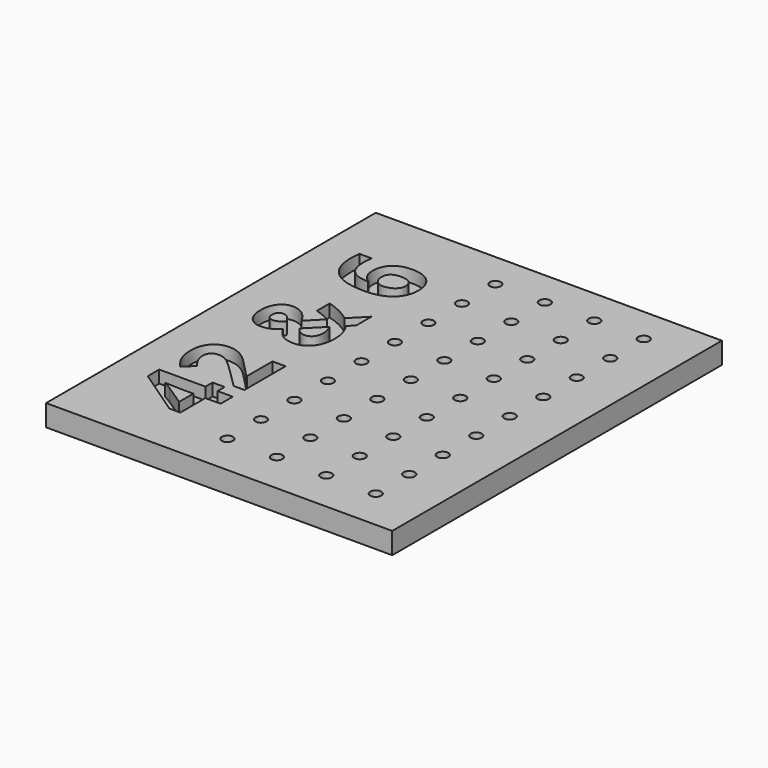
from build123d import *

# Parameters (mm, degrees)
F0_W         = 42
F0_H         = 50
F1_DEPTH     = 2.6
F2_TEXT_SIZE = 12.5
F3_DEPTH     = 1.5
F4_R         = 0.675
F5_DEPTH     = 2.6


# Not quite as in the source:
# - Text() gives the source's letters only with a copy of the font that has no kerning and outlines rounded to 1/6400 em; it was checked with that copy


with BuildPart() as f1:
    # F0 (on Top) → F1 (new body)
    with BuildSketch(Plane.XY):
        with Locations((-22.1587231159, 3.3350909071)):
            Rectangle(F0_W, F0_H)
    extrude(amount=F1_DEPTH)

    # F2 (on face) → F3 (cut)
    with BuildSketch(Plane.XY.offset(2.6)):
        with Locations(Location((-30.1587231159, -15.4649090929), (0, 0, 90))):
            Text('42 & 6', F2_TEXT_SIZE, font='Open Sans', font_style=FontStyle.BOLD, text_align=(TextAlign.LEFT, TextAlign.BOTTOM))
    extrude(amount=-F3_DEPTH, mode=Mode.SUBTRACT)

    # F4 (on face) → F5 (cut, through all)
    with BuildSketch(Plane.XY.offset(2.6)):
        with Locations((-25.1587231159, -16.6649090929)):
            Circle(F4_R)
        with Locations((-25.1587231159, -11.5849090929)):
            Circle(F4_R)
        with Locations((-25.1587231159, -6.5049090929)):
            Circle(F4_R)
        with Locations((-25.1587231159, -1.4249090929)):
            Circle(F4_R)
        with Locations((-25.1587231159, 3.6550909071)):
            Circle(F4_R)
        with Locations((-25.1587231159, 8.7350909071)):
            Circle(F4_R)
        with Locations((-25.1587231159, 13.8150909071)):
            Circle(F4_R)
        with Locations((-25.1587231159, 18.8950909071)):
            Circle(F4_R)
        with Locations((-19.1587231159, -16.6649090929)):
            Circle(F4_R)
        with Locations((-19.1587231159, -11.5849090929)):
            Circle(F4_R)
        with Locations((-19.1587231159, -6.5049090929)):
            Circle(F4_R)
        with Locations((-19.1587231159, -1.4249090929)):
            Circle(F4_R)
        with Locations((-19.1587231159, 3.6550909071)):
            Circle(F4_R)
        with Locations((-19.1587231159, 8.7350909071)):
            Circle(F4_R)
        with Locations((-19.1587231159, 13.8150909071)):
            Circle(F4_R)
        with Locations((-19.1587231159, 18.8950909071)):
            Circle(F4_R)
        with Locations((-13.1587231159, -16.6649090929)):
            Circle(F4_R)
        with Locations((-13.1587231159, -11.5849090929)):
            Circle(F4_R)
        with Locations((-13.1587231159, -6.5049090929)):
            Circle(F4_R)
        with Locations((-13.1587231159, -1.4249090929)):
            Circle(F4_R)
        with Locations((-13.1587231159, 3.6550909071)):
            Circle(F4_R)
        with Locations((-13.1587231159, 8.7350909071)):
            Circle(F4_R)
        with Locations((-13.1587231159, 13.8150909071)):
            Circle(F4_R)
        with Locations((-13.1587231159, 18.8950909071)):
            Circle(F4_R)
        with Locations((-25.1587231159, 23.9750909071)):
            Circle(F4_R)
        with Locations((-19.1587231159, 23.9750909071)):
            Circle(F4_R)
        with Locations((-13.1587231159, 23.9750909071)):
            Circle(F4_R)
        with Locations((-7.1587231159, -16.6649090929)):
            Circle(F4_R)
        with Locations((-7.1587231159, -11.5849090929)):
            Circle(F4_R)
        with Locations((-7.1587231159, -6.5049090929)):
            Circle(F4_R)
        with Locations((-7.1587231159, -1.4249090929)):
            Circle(F4_R)
        with Locations((-7.1587231159, 3.6550909071)):
            Circle(F4_R)
        with Locations((-7.1587231159, 8.7350909071)):
            Circle(F4_R)
        with Locations((-7.1587231159, 13.8150909071)):
            Circle(F4_R)
        with Locations((-7.1587231159, 18.8950909071)):
            Circle(F4_R)
        with Locations((-7.1587231159, 23.9750909071)):
            Circle(F4_R)
    extrude(amount=-F5_DEPTH, mode=Mode.SUBTRACT)


solid = f1.part
